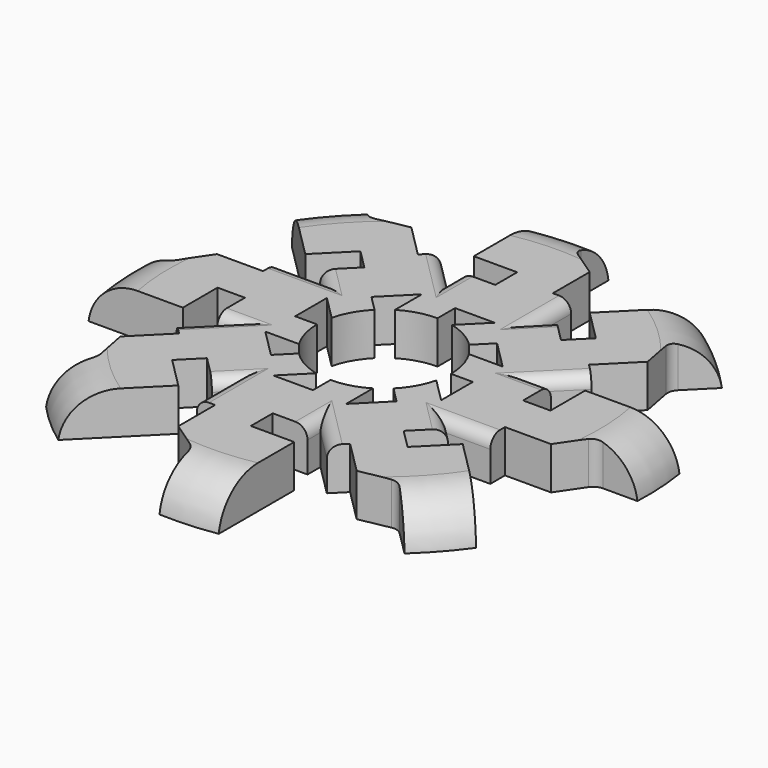
from build123d import *

# Parameters (mm, degrees)
F2_DEPTH     = 7
F3_T2_ANGLE  = 61.2363952851
F4_T2_ANGLE  = 61.2363952851
F4_T4_ANGLE  = 61.2363952851
F4_T6_ANGLE  = 61.2363952851
F4_T8_ANGLE  = 61.2363952851
F4_T10_ANGLE = 61.2363952851
F4_T12_ANGLE = 61.2363952851
F4_T14_ANGLE = 61.2363952851
F5_R         = 2
F6_R         = 2


# Not quite as in the source:
# - a fillet or chamfer that OpenCascade refuses, or shapes differently, is made with other operations: its cross-section is extruded or revolved along the edge and cut away or added


with BuildPart() as f2:
    # F1 (on Top) → F2 (new body)
    with BuildSketch(Plane.XY):
        with BuildLine():
            Line((0, 27.3689869791), (0, 22.8657480371))
            Line((0, 22.8657480371), (-5.7183573954, 22.8657480371))
            Line((-5.7183573954, 22.8657480371), (-5.7183573954, 20.2005400622))
            Line((-5.7183573954, 20.2005400622), (-3.0870979442, 17.5692806111))
            Line((-3.0870979442, 17.5692806111), (-5.7183573954, 14.9380211599))
            Line((-5.7183573954, 14.9380211599), (-5.7183573954, 9.3968286511))
            ThreePointArc((-5.7183573954, 9.3968286511), (-2.9694178586, 10.5916267675), (0, 11))
            Line((0, 11), (0, 14.6062653512))
            Line((0, 14.6062653512), (6.5192867681, 14.6062653512))
            Line((6.5192867681, 14.6062653512), (10.2404495701, 18.3274281532))
            Line((10.2404495701, 18.3274281532), (10.2404495701, 25.6717079897))
            Line((10.2404495701, 25.6717079897), (7.2286586717, 25.6717079897))
            Line((7.2286586717, 25.6717079897), (7.2286586717, 33.2464904108))
            Line((7.2286586717, 33.2464904108), (2.1756596398, 36.6748697717))
            Line((2.1756596398, 36.6748697717), (2.1756596398, 43.4126186022))
            ThreePointArc((2.1756596398, 43.4126186022), (-2.4920924901, 43.3788722548), (-7.132247556, 42.8709256758))
            Line((-7.132247556, 42.8709256758), (-7.132247556, 27.3689869791))
            Line((-7.132247556, 27.3689869791), (0, 27.3689869791))
        make_face()
        Polygon((-3.0870979442, 17.5692806111), (-5.7183573954, 20.2005400622), (-5.7183573954, 14.9380211599), align=None)
        with BuildLine():
            Line((-5.7183573954, 14.9380211599), (-5.7183573954, 20.2005400622))
            Line((-5.7183573954, 20.2005400622), (-10.9115474707, 25.3937301376))
            Line((-10.9115474707, 25.3937301376), (-13.0412052386, 23.2640723698))
            Line((-13.0412052386, 23.2640723698), (-18.3973852545, 28.6202523857))
            Line((-18.3973852545, 28.6202523857), (-24.3946254299, 27.4714727995))
            Line((-24.3946254299, 27.4714727995), (-29.1589333179, 32.2357806875))
            ThreePointArc((-29.1589333179, 32.2357806875), (-32.4356702307, 28.9113192324), (-35.3575828731, 25.2710616492))
            Line((-35.3575828731, 25.2710616492), (-24.3960568991, 14.3095356752))
            Line((-24.3960568991, 14.3095356752), (-19.3527962871, 19.3527962871))
            Line((-19.3527962871, 19.3527962871), (-16.1685254939, 16.1685254939))
            Line((-16.1685254939, 16.1685254939), (-20.2120147854, 12.1250362024))
            Line((-20.2120147854, 12.1250362024), (-18.3274281532, 10.2404495701))
            Line((-18.3274281532, 10.2404495701), (-14.6062653512, 10.2404495701))
            Line((-14.6062653512, 10.2404495701), (-14.6062653512, 6.5192867681))
            Line((-14.6062653512, 6.5192867681), (-10.6880505524, 2.6010719693))
            ThreePointArc((-10.6880505524, 2.6010719693), (-9.589106615, 5.3897156071), (-7.7781745931, 7.7781745931))
            Line((-7.7781745931, 7.7781745931), (-10.3281892776, 10.3281892776))
            Line((-10.3281892776, 10.3281892776), (-5.7183573954, 14.9380211599))
        make_face()
        Polygon((10.2404495701, 18.3274281532), (6.5192867681, 14.6062653512), (10.2404495701, 14.6062653512), align=None)
        with BuildLine():
            Line((10.2404495701, 14.6062653512), (6.5192867681, 14.6062653512))
            Line((6.5192867681, 14.6062653512), (2.6010719693, 10.6880505524))
            ThreePointArc((2.6010719693, 10.6880505524), (5.3897156071, 9.589106615), (7.7781745931, 7.7781745931))
            Line((7.7781745931, 7.7781745931), (10.3281892776, 10.3281892776))
            Line((10.3281892776, 10.3281892776), (14.9380211599, 5.7183573954))
            Line((14.9380211599, 5.7183573954), (20.2005400622, 5.7183573954))
            Line((20.2005400622, 5.7183573954), (25.3937301376, 10.9115474707))
            Line((25.3937301376, 10.9115474707), (23.2640723698, 13.0412052386))
            Line((23.2640723698, 13.0412052386), (28.6202523857, 18.3973852545))
            Line((28.6202523857, 18.3973852545), (27.4714727995, 24.3946254299))
            Line((27.4714727995, 24.3946254299), (32.2357806875, 29.1589333179))
            ThreePointArc((32.2357806875, 29.1589333179), (28.9113192324, 32.4356702307), (25.2710616492, 35.3575828731))
            Line((25.2710616492, 35.3575828731), (14.3095356752, 24.3960568991))
            Line((14.3095356752, 24.3960568991), (19.3527962871, 19.3527962871))
            Line((19.3527962871, 19.3527962871), (16.1685254939, 16.1685254939))
            Line((16.1685254939, 16.1685254939), (12.1250362024, 20.2120147854))
            Line((12.1250362024, 20.2120147854), (10.2404495701, 18.3274281532))
            Line((10.2404495701, 18.3274281532), (10.2404495701, 14.6062653512))
        make_face()
        with BuildLine():
            Line((-14.6062653512, 0), (-14.6062653512, 6.5192867681))
            Line((-14.6062653512, 6.5192867681), (-18.3274281532, 10.2404495701))
            Line((-18.3274281532, 10.2404495701), (-25.6717079897, 10.2404495701))
            Line((-25.6717079897, 10.2404495701), (-25.6717079897, 7.2286586717))
            Line((-25.6717079897, 7.2286586717), (-33.2464904108, 7.2286586717))
            Line((-33.2464904108, 7.2286586717), (-36.6748697717, 2.1756596398))
            Line((-36.6748697717, 2.1756596398), (-43.4126186022, 2.1756596398))
            ThreePointArc((-43.4126186022, 2.1756596398), (-43.3788722548, -2.4920924901), (-42.8709256758, -7.132247556))
            Line((-42.8709256758, -7.132247556), (-27.3689869791, -7.132247556))
            Line((-27.3689869791, -7.132247556), (-27.3689869791, 0))
            Line((-27.3689869791, 0), (-22.8657480371, 0))
            Line((-22.8657480371, 0), (-22.8657480371, -5.7183573954))
            Line((-22.8657480371, -5.7183573954), (-20.2005400622, -5.7183573954))
            Line((-20.2005400622, -5.7183573954), (-17.5692806111, -3.0870979442))
            Line((-17.5692806111, -3.0870979442), (-14.9380211599, -5.7183573954))
            Line((-14.9380211599, -5.7183573954), (-9.3968286511, -5.7183573954))
            ThreePointArc((-9.3968286511, -5.7183573954), (-10.5916267675, -2.9694178586), (-11, 0))
            Line((-11, 0), (-14.6062653512, 0))
        make_face()
        Polygon((-18.3274281532, 10.2404495701), (-14.6062653512, 6.5192867681), (-14.6062653512, 10.2404495701), align=None)
        with BuildLine():
            Line((17.5692806111, 3.0870979442), (14.9380211599, 5.7183573954))
            Line((14.9380211599, 5.7183573954), (9.3968286511, 5.7183573954))
            ThreePointArc((9.3968286511, 5.7183573954), (10.5916267675, 2.9694178586), (11, 0))
            Line((11, 0), (14.6062653512, 0))
            Line((14.6062653512, 0), (14.6062653512, -6.5192867681))
            Line((14.6062653512, -6.5192867681), (18.3274281532, -10.2404495701))
            Line((18.3274281532, -10.2404495701), (25.6717079897, -10.2404495701))
            Line((25.6717079897, -10.2404495701), (25.6717079897, -7.2286586717))
            Line((25.6717079897, -7.2286586717), (33.2464904108, -7.2286586717))
            Line((33.2464904108, -7.2286586717), (36.6748697717, -2.1756596398))
            Line((36.6748697717, -2.1756596398), (43.4126186022, -2.1756596398))
            ThreePointArc((43.4126186022, -2.1756596398), (43.3788722548, 2.4920924901), (42.8709256758, 7.132247556))
            Line((42.8709256758, 7.132247556), (27.3689869791, 7.132247556))
            Line((27.3689869791, 7.132247556), (27.3689869791, 0))
            Line((27.3689869791, 0), (22.8657480371, 0))
            Line((22.8657480371, 0), (22.8657480371, 5.7183573954))
            Line((22.8657480371, 5.7183573954), (20.2005400622, 5.7183573954))
            Line((20.2005400622, 5.7183573954), (17.5692806111, 3.0870979442))
        make_face()
        Polygon((20.2005400622, 5.7183573954), (14.9380211599, 5.7183573954), (17.5692806111, 3.0870979442), align=None)
        with BuildLine():
            Line((-10.3281892776, -10.3281892776), (-14.9380211599, -5.7183573954))
            Line((-14.9380211599, -5.7183573954), (-20.2005400622, -5.7183573954))
            Line((-20.2005400622, -5.7183573954), (-25.3937301376, -10.9115474707))
            Line((-25.3937301376, -10.9115474707), (-23.2640723698, -13.0412052386))
            Line((-23.2640723698, -13.0412052386), (-28.6202523857, -18.3973852545))
            Line((-28.6202523857, -18.3973852545), (-27.4714727995, -24.3946254299))
            Line((-27.4714727995, -24.3946254299), (-32.2357806875, -29.1589333179))
            ThreePointArc((-32.2357806875, -29.1589333179), (-28.9113192324, -32.4356702307), (-25.2710616492, -35.3575828731))
            Line((-25.2710616492, -35.3575828731), (-14.3095356752, -24.3960568991))
            Line((-14.3095356752, -24.3960568991), (-19.3527962871, -19.3527962871))
            Line((-19.3527962871, -19.3527962871), (-16.1685254939, -16.1685254939))
            Line((-16.1685254939, -16.1685254939), (-12.1250362024, -20.2120147854))
            Line((-12.1250362024, -20.2120147854), (-10.2404495701, -18.3274281532))
            Line((-10.2404495701, -18.3274281532), (-10.2404495701, -14.6062653512))
            Line((-10.2404495701, -14.6062653512), (-6.5192867681, -14.6062653512))
            Line((-6.5192867681, -14.6062653512), (-2.6010719693, -10.6880505524))
            ThreePointArc((-2.6010719693, -10.6880505524), (-5.3897156071, -9.589106615), (-7.7781745931, -7.7781745931))
            Line((-7.7781745931, -7.7781745931), (-10.3281892776, -10.3281892776))
        make_face()
        Polygon((-20.2005400622, -5.7183573954), (-14.9380211599, -5.7183573954), (-17.5692806111, -3.0870979442), align=None)
        with BuildLine():
            Line((14.6062653512, -10.2404495701), (14.6062653512, -6.5192867681))
            Line((14.6062653512, -6.5192867681), (10.6880505524, -2.6010719693))
            ThreePointArc((10.6880505524, -2.6010719693), (9.589106615, -5.3897156071), (7.7781745931, -7.7781745931))
            Line((7.7781745931, -7.7781745931), (10.3281892776, -10.3281892776))
            Line((10.3281892776, -10.3281892776), (5.7183573954, -14.9380211599))
            Line((5.7183573954, -14.9380211599), (5.7183573954, -20.2005400622))
            Line((5.7183573954, -20.2005400622), (10.9115474707, -25.3937301376))
            Line((10.9115474707, -25.3937301376), (13.0412052386, -23.2640723698))
            Line((13.0412052386, -23.2640723698), (18.3973852545, -28.6202523857))
            Line((18.3973852545, -28.6202523857), (24.3946254299, -27.4714727995))
            Line((24.3946254299, -27.4714727995), (29.1589333179, -32.2357806875))
            ThreePointArc((29.1589333179, -32.2357806875), (32.4356702307, -28.9113192324), (35.3575828731, -25.2710616492))
            Line((35.3575828731, -25.2710616492), (24.3960568991, -14.3095356752))
            Line((24.3960568991, -14.3095356752), (19.3527962871, -19.3527962871))
            Line((19.3527962871, -19.3527962871), (16.1685254939, -16.1685254939))
            Line((16.1685254939, -16.1685254939), (20.2120147854, -12.1250362024))
            Line((20.2120147854, -12.1250362024), (18.3274281532, -10.2404495701))
            Line((18.3274281532, -10.2404495701), (14.6062653512, -10.2404495701))
        make_face()
        Polygon((18.3274281532, -10.2404495701), (14.6062653512, -6.5192867681), (14.6062653512, -10.2404495701), align=None)
        with BuildLine():
            Line((0, -14.6062653512), (-6.5192867681, -14.6062653512))
            Line((-6.5192867681, -14.6062653512), (-10.2404495701, -18.3274281532))
            Line((-10.2404495701, -18.3274281532), (-10.2404495701, -25.6717079897))
            Line((-10.2404495701, -25.6717079897), (-7.2286586717, -25.6717079897))
            Line((-7.2286586717, -25.6717079897), (-7.2286586717, -33.2464904108))
            Line((-7.2286586717, -33.2464904108), (-2.1756596398, -36.6748697717))
            Line((-2.1756596398, -36.6748697717), (-2.1756596398, -43.4126186022))
            ThreePointArc((-2.1756596398, -43.4126186022), (2.4920924901, -43.3788722548), (7.132247556, -42.8709256758))
            Line((7.132247556, -42.8709256758), (7.132247556, -27.3689869791))
            Line((7.132247556, -27.3689869791), (0, -27.3689869791))
            Line((0, -27.3689869791), (0, -22.8657480371))
            Line((0, -22.8657480371), (5.7183573954, -22.8657480371))
            Line((5.7183573954, -22.8657480371), (5.7183573954, -20.2005400622))
            Line((5.7183573954, -20.2005400622), (3.0870979442, -17.5692806111))
            Line((3.0870979442, -17.5692806111), (5.7183573954, -14.9380211599))
            Line((5.7183573954, -14.9380211599), (5.7183573954, -9.3968286511))
            ThreePointArc((5.7183573954, -9.3968286511), (2.9694178586, -10.5916267675), (0, -11))
            Line((0, -11), (0, -14.6062653512))
        make_face()
        Polygon((-10.2404495701, -18.3274281532), (-6.5192867681, -14.6062653512), (-10.2404495701, -14.6062653512), align=None)
        Polygon((5.7183573954, -20.2005400622), (5.7183573954, -14.9380211599), (3.0870979442, -17.5692806111), align=None)
    extrude(amount=F2_DEPTH)

    # F3: fillet of radius 8 on 1 edges, made by hand

    # F3_s1 → F3_t2 (revolve, cut)
    with BuildSketch(Plane(origin=(-0.3836282994, 1.2011620881, 0), x_dir=(0, 0, 1), z_dir=(-0.3042407592, 0.9525951713, 0))):
        with BuildLine():
            ThreePointArc((0, -43.8044169447), (5, -41.1586656337), (7, -35.8671630115))
            Line((7, -35.8671630115), (7, -43.8044169447))
            Line((7, -43.8044169447), (0, -43.8044169447))
        make_face()
    revolve(axis=Axis((1.5854000596, 1.8300322534, 7), (0, 0, 1)), revolution_arc=F3_T2_ANGLE, mode=Mode.SUBTRACT)

    # F4: fillet of radius 8 on 7 edges, made by hand

    # F4_s1 → F4_t2 (revolve, cut)
    with BuildSketch(Plane(origin=(-1.2011620881, -0.3836282994, 0), x_dir=(0, 0, 1), z_dir=(-0.9525951713, -0.3042407592, 0))):
        with BuildLine():
            ThreePointArc((7, -35.8671630115), (5, -41.1586656337), (0, -43.8044169447))
            Line((0, -43.8044169447), (7, -43.8044169447))
            Line((7, -43.8044169447), (7, -35.8671630115))
        make_face()
    revolve(axis=Axis((-1.8300322534, 1.5854000596, 7), (0, 0, 1)), revolution_arc=F4_T2_ANGLE, mode=Mode.SUBTRACT)

    # F4_s3 → F4_t4 (revolve, cut)
    with BuildSketch(Plane(origin=(-1.1206160298, 0.5780836858, 0), x_dir=(0, 0, 1), z_dir=(-0.8887172093, 0.4584558014, 0))):
        with BuildLine():
            ThreePointArc((7, -35.8671630115), (5, -41.1586656337), (0, -43.8044169447))
            Line((0, -43.8044169447), (7, -43.8044169447))
            Line((7, -43.8044169447), (7, -35.8671630115))
        make_face()
    revolve(axis=Axis((-0.1729810831, 2.4150753492, 7), (0, 0, 1)), revolution_arc=F4_T4_ANGLE, mode=Mode.SUBTRACT)

    # F4_s5 → F4_t6 (revolve, cut)
    with BuildSketch(Plane(origin=(-0.5780836858, -1.1206160298, 0), x_dir=(0, 0, 1), z_dir=(-0.4584558014, -0.8887172093, 0))):
        with BuildLine():
            ThreePointArc((7, -35.8671630115), (5, -41.1586656337), (0, -43.8044169447))
            Line((0, -43.8044169447), (7, -43.8044169447))
            Line((7, -43.8044169447), (7, -35.8671630115))
        make_face()
    revolve(axis=Axis((-2.4150753492, -0.1729810831, 7), (0, 0, 1)), revolution_arc=F4_T6_ANGLE, mode=Mode.SUBTRACT)

    # F4_s7 → F4_t8 (revolve, cut)
    with BuildSketch(Plane(origin=(0.3836282994, -1.2011620881, 0), x_dir=(0, 0, 1), z_dir=(0.3042407592, -0.9525951713, 0))):
        with BuildLine():
            ThreePointArc((7, -35.8671630115), (5, -41.1586656337), (0, -43.8044169447))
            Line((0, -43.8044169447), (7, -43.8044169447))
            Line((7, -43.8044169447), (7, -35.8671630115))
        make_face()
    revolve(axis=Axis((-1.5854000596, -1.8300322534, 7), (0, 0, 1)), revolution_arc=F4_T8_ANGLE, mode=Mode.SUBTRACT)

    # F4_s9 → F4_t10 (revolve, cut)
    with BuildSketch(Plane(origin=(1.1206160298, -0.5780836858, 0), x_dir=(0, 0, 1), z_dir=(0.8887172093, -0.4584558014, 0))):
        with BuildLine():
            ThreePointArc((7, -35.8671630115), (5, -41.1586656337), (0, -43.8044169447))
            Line((0, -43.8044169447), (7, -43.8044169447))
            Line((7, -43.8044169447), (7, -35.8671630115))
        make_face()
    revolve(axis=Axis((0.1729810831, -2.4150753492, 7), (0, 0, 1)), revolution_arc=F4_T10_ANGLE, mode=Mode.SUBTRACT)

    # F4_s11 → F4_t12 (revolve, cut)
    with BuildSketch(Plane(origin=(1.2011620881, 0.3836282994, 0), x_dir=(0, 0, 1), z_dir=(0.9525951713, 0.3042407592, 0))):
        with BuildLine():
            ThreePointArc((7, -35.8671630115), (5, -41.1586656337), (0, -43.8044169447))
            Line((0, -43.8044169447), (7, -43.8044169447))
            Line((7, -43.8044169447), (7, -35.8671630115))
        make_face()
    revolve(axis=Axis((1.8300322534, -1.5854000596, 7), (0, 0, 1)), revolution_arc=F4_T12_ANGLE, mode=Mode.SUBTRACT)

    # F4_s13 → F4_t14 (revolve, cut)
    with BuildSketch(Plane(origin=(0.5780836858, 1.1206160298, 0), x_dir=(0, 0, 1), z_dir=(0.4584558014, 0.8887172093, 0))):
        with BuildLine():
            ThreePointArc((7, -35.8671630115), (5, -41.1586656337), (0, -43.8044169447))
            Line((0, -43.8044169447), (7, -43.8044169447))
            Line((7, -43.8044169447), (7, -35.8671630115))
        make_face()
    revolve(axis=Axis((2.4150753492, 0.1729810831, 7), (0, 0, 1)), revolution_arc=F4_T14_ANGLE, mode=Mode.SUBTRACT)

    # F5
    f5_edges = [f2.edges().sort_by_distance(p)[0] for p in [
        (21.533144, 5.718357, 7),
        (22.797135, 8.314952, 7),
        (10.24045, 21.999568, 7),
        (11.182743, 19.269721, 7),
        (-8.314952, 22.797135, 7),
        (-5.718357, 21.533144, 7),
        (-21.999568, 10.24045, 7),
        (-19.269721, 11.182743, 7),
        (-22.797135, -8.314952, 7),
        (-21.533144, -5.718357, 7),
        (-11.182743, -19.269721, 7),
        (-10.24045, -21.999568, 7),
        (5.718357, -21.533144, 7),
        (8.314952, -22.797135, 7),
        (21.999568, -10.24045, 7),
        (19.269721, -11.182743, 7),
    ]]
    fillet(f5_edges, radius=F5_R)

    # F6
    f6_edges = [f2.edges().sort_by_distance(p)[0] for p in [
        (-36.67487, 2.17566, 3.454209),
        (-24.394625, 27.471473, 3.454209),
        (2.17566, 36.67487, 3.454209),
        (27.471473, 24.394625, 3.454209),
        (36.67487, -2.17566, 3.454209),
        (24.394625, -27.471473, 3.454209),
        (-2.17566, -36.67487, 3.454209),
        (-27.471473, -24.394625, 3.454209),
    ]]
    fillet(f6_edges, radius=F6_R)


solid = f2.part
